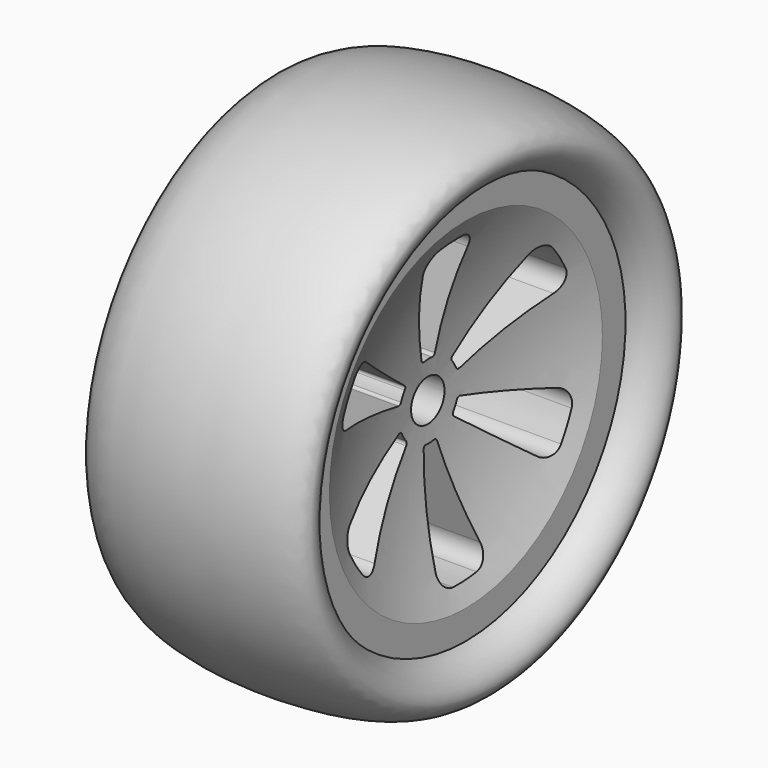
from build123d import *

# Parameters (mm, degrees)
F5_DEPTH        = 81.7343349895
F5_COPIES_COUNT = 6
F6_R            = 8.7631837749
F7_DEPTH        = 46.6975364229
F7_DEPTH_BACK   = 47.6213796249


# Not quite as in the source:
# - a pattern or mirror of a feature is missing from the dataset's text; its kind, count and spacing are read off the source's solid


with BuildPart() as f1:
    # F0 (on Front) → F1 (revolve)
    with BuildSketch(Plane.XZ):
        with BuildLine():
            add(Edge.make_bspline(
                [(-45.9521748126, 59.689514339), (-41.9680401638, 67.8841583445), (-0.4836835479, 74.7989063149), (56.6748879922, 65.7053778676), (37.8451563684, 39.802802976), (0.541377707, 53.4771669982), (-40.6494688889, 39.3845085448), (-48.1295824117, 55.2109809302), (-45.9521748126, 59.689514339)],
                knots=[0, 0, 0, 0, 0.2018973944, 0.4063785635, 0.5218312028, 0.7040180019, 0.8896591206, 1, 1, 1, 1], degree=3))
        make_face()
    revolve(axis=Axis((0.0194367021, 0, -37.7883389592), (-1, 0, 0)))


with BuildPart() as f3:
    # F2 (on Front) → F3 (revolve)
    with BuildSketch(Plane.XZ):
        with BuildLine():
            Line((35.0367985666, 46.9480757509), (-38.9862209558, 46.9480757509))
            Line((-38.9862209558, 46.9480757509), (-38.9862209558, 33.1435985863))
            ThreePointArc((-38.9862209558, 33.1435985863), (-29.5389908092, -1.7646134017), (-26.3570702245, -37.7883389592))
            Line((-26.3570702245, -37.7883389592), (18.8512488193, -37.7883389592))
            ThreePointArc((18.8512488193, -37.7883389592), (22.9481431001, -1.1181309847), (35.0367985666, 33.7437838316))
            Line((35.0367985666, 33.7437838316), (35.0367985666, 46.9480757509))
        make_face()
    revolve(axis=Axis((0.0194367021, 0, -37.7883389592), (-1, 0, 0)))

    # F4 (on face) → F5 (cut, through all)
    with BuildSketch(Plane.YZ.offset(35.0367985666)):
        with BuildLine():
            Line((-15.0041714376, 17.4010789654), (-4.0817300079, -21.4959818709))
            ThreePointArc((-4.0817300079, -21.4959818709), (-3.5373061157, -22.2263396529), (-2.6439118694, -22.4042907276))
            ThreePointArc((-2.6439118694, -22.4042907276), (-0.5488930929, -22.1884054229), (1.5561180441, -22.2565101359))
            ThreePointArc((1.5561180441, -22.2565101359), (2.4684254273, -21.9906209115), (2.9408483482, -21.1661098898))
            Line((2.9408483482, -21.1661098898), (8.4590197059, 18.9009046542))
            ThreePointArc((8.4590197059, 18.9009046542), (7.0327540045, 23.8490049937), (2.4074646907, 26.1127694655))
            ThreePointArc((2.4074646907, 26.1127694655), (-3.7490537223, 26.0481094095), (-9.8708179469, 25.3916776378))
            ThreePointArc((-9.8708179469, 25.3916776378), (-14.2331628133, 22.5499588523), (-15.0041714376, 17.4010789654))
        make_face()
    f5 = extrude(amount=-F5_DEPTH, mode=Mode.SUBTRACT)

    # F5_copies: F5 ×6 about axis
    f5_copies_axis = Axis((0, 0, -37.788339), (1, 0, 0))
    for i in range(1, F5_COPIES_COUNT):
        add(f5.rotate(f5_copies_axis, i * 360 / F5_COPIES_COUNT), mode=Mode.SUBTRACT)

    # F6 (on Right) → F7 (cut, two sides)
    with BuildSketch(Plane.YZ) as f7_sk:
        with Locations((0, -37.7883389592)):
            Circle(F6_R)
    extrude(amount=-F7_DEPTH, mode=Mode.SUBTRACT)
    extrude(f7_sk.sketch, amount=F7_DEPTH_BACK, mode=Mode.SUBTRACT)


solid = Compound([f1.part, f3.part])
